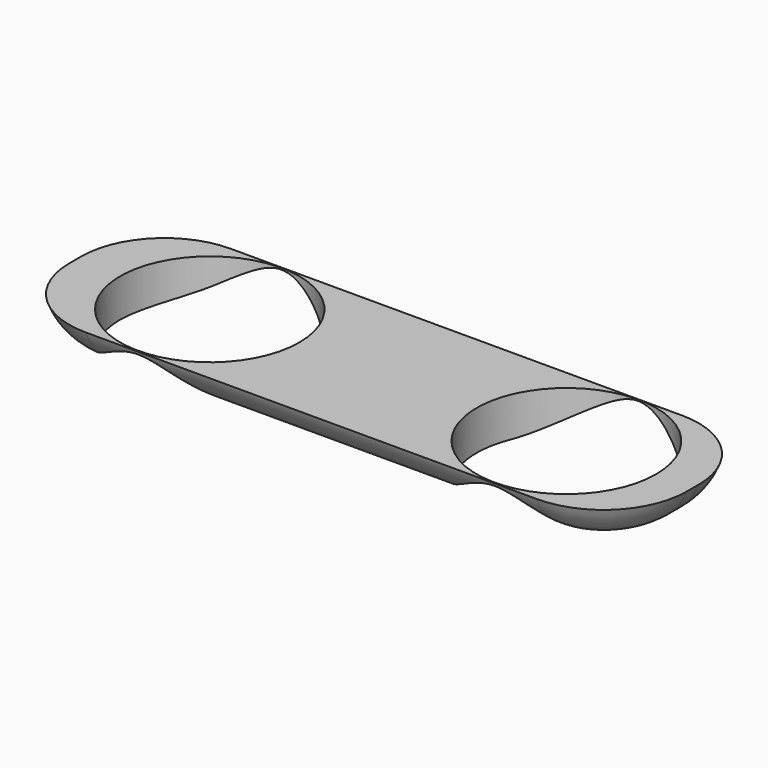
from build123d import *

# Parameters (mm, degrees)
F0_R         = 25.3224131448
F0_R_2       = 25.3609127301
F1_DEPTH     = 11.176
F2_T1_DEPTH  = 4.1998379789
F2_T3_DEPTH  = 127.4783204379
F2_T5_DEPTH  = 4.1998416744
F2_T7_DEPTH  = 127.4783167424
F2_T10_ANGLE = 90
F2_T12_ANGLE = 90
F2_T14_ANGLE = 90
F2_T16_ANGLE = 90


# Not quite as in the source:
# - a fillet or chamfer that OpenCascade refuses, or shapes differently, is made with other operations: its cross-section is extruded or revolved along the edge and cut away or added


with BuildPart() as f1:
    # F0 (on Top) → F1 (new body)
    with BuildSketch(Plane.XY):
        with BuildLine():
            Line((70.0572131213, 37.4184697866), (-57.4211036211, 37.4184697866))
            ThreePointArc((-57.4211036211, 37.4184697866), (-74.0383517658, 30.5353802358), (-80.9214413166, 13.9181320912))
            Line((-80.9214413166, 13.9181320912), (-80.9214413166, 9.7182941123))
            ThreePointArc((-80.9214413166, 9.7182941123), (-74.0383528482, -6.8989514193), (-57.4211073166, -13.7820398877))
            Line((-57.4211073166, -13.7820398877), (70.0572131213, -13.7820398877))
            ThreePointArc((70.0572131213, -13.7820398877), (86.6744586529, -6.8989514193), (93.5575471213, 9.7182941123))
            Line((93.5575471213, 9.7182941123), (93.5575471213, 13.9181357866))
            ThreePointArc((93.5575471213, 13.9181357866), (86.6744586529, 30.5353813182), (70.0572131213, 37.4184697866))
        make_face()
        with Locations((-42.9976209998, 11.9247278199)):
            Circle(F0_R, mode=Mode.SUBTRACT)
        with Locations((57.7639937401, 11.9247278199)):
            Circle(F0_R_2, mode=Mode.SUBTRACT)
    extrude(amount=F1_DEPTH)

    # F2: fillet of radius 17.1698868556 on 1 edges, made by hand

    # F2_s2 → F2_t1 (cut)
    with BuildSketch(Plane.XZ.offset(-13.9181320912)):
        with BuildLine():
            ThreePointArc((-80.9214413166, 11.176), (-74.6269133611, 3.0681250194), (-64.8317447689, 0))
            Line((-64.8317447689, 0), (-64.8317447689, -0.3433977371))
            Line((-64.8317447689, -0.3433977371), (-80.9214413166, -0.3433977371))
            Line((-80.9214413166, -0.3433977371), (-81.2648390537, 0))
            ThreePointArc((-81.2648390537, 0), (-81.2648390537, 5.588), (-81.2432352476, 11.0561222629))
            Line((-81.2432352476, 11.0561222629), (-80.9214413166, 11.176))
        make_face()
    extrude(amount=F2_T1_DEPTH, mode=Mode.SUBTRACT)

    # F2_s4 → F2_t3 (cut)
    with BuildSketch(Plane.YZ.offset(-57.4211073166)):
        with BuildLine():
            ThreePointArc((-13.7820398877, 11.176), (-7.4875119322, 3.0681250194), (2.3076566599, 0))
            Line((2.3076566599, 0), (2.3076566599, -0.3433977371))
            Line((2.3076566599, -0.3433977371), (-13.7820398877, -0.3433977371))
            Line((-13.7820398877, -0.3433977371), (-14.1254376248, 0))
            ThreePointArc((-14.1254376248, 0), (-14.1254376248, 5.588), (-14.1038338187, 11.0561222629))
            Line((-14.1038338187, 11.0561222629), (-13.7820398877, 11.176))
        make_face()
    extrude(amount=F2_T3_DEPTH, mode=Mode.SUBTRACT)

    # F2_s6 → F2_t5 (cut)
    with BuildSketch(Plane.XZ.offset(-13.9181357866)):
        with BuildLine():
            ThreePointArc((93.5575471213, 11.176), (87.2630191658, 3.0681250194), (77.4678505736, 0))
            Line((77.4678505736, 0), (77.4678505736, -0.3433977371))
            Line((77.4678505736, -0.3433977371), (93.5575471213, -0.3433977371))
            Line((93.5575471213, -0.3433977371), (93.9009448584, 0))
            ThreePointArc((93.9009448584, 0), (93.9009448584, 5.588), (93.8793410523, 11.0561222629))
            Line((93.8793410523, 11.0561222629), (93.5575471213, 11.176))
        make_face()
    extrude(amount=F2_T5_DEPTH, mode=Mode.SUBTRACT)

    # F2_s8 → F2_t7 (cut)
    with BuildSketch(Plane.YZ.offset(-57.4211036211)):
        with BuildLine():
            ThreePointArc((37.4184697866, 11.176), (31.1239418311, 3.0681250194), (21.328773239, 0))
            Line((21.328773239, 0), (21.328773239, -0.3433977371))
            Line((21.328773239, -0.3433977371), (37.4184697866, -0.3433977371))
            Line((37.4184697866, -0.3433977371), (37.7618675238, 0))
            ThreePointArc((37.7618675238, 0), (37.7618675238, 5.588), (37.7402637176, 11.0561222629))
            Line((37.7402637176, 11.0561222629), (37.4184697866, 11.176))
        make_face()
    extrude(amount=F2_T7_DEPTH, mode=Mode.SUBTRACT)

    # F2_s9 → F2_t10 (revolve, cut)
    with BuildSketch(Plane.XZ.offset(-9.7182941123)):
        with BuildLine():
            ThreePointArc((-80.9214413166, 11.176), (-74.6269133611, 3.0681250194), (-64.8317447689, 0))
            Line((-64.8317447689, 0), (-64.8317447689, -0.3433977371))
            Line((-64.8317447689, -0.3433977371), (-80.9214413166, -0.3433977371))
            Line((-80.9214413166, -0.3433977371), (-81.2648390537, 0))
            ThreePointArc((-81.2648390537, 0), (-81.2648390537, 5.588), (-81.2432352476, 11.0561222629))
            Line((-81.2432352476, 11.0561222629), (-80.9214413166, 11.176))
        make_face()
    revolve(axis=Axis((-57.4211073166, 9.7182941123, 0), (0, 0, 1)), revolution_arc=F2_T10_ANGLE, mode=Mode.SUBTRACT)

    # F2_s11 → F2_t12 (revolve, cut)
    with BuildSketch(Plane.YZ.offset(70.0572131213)):
        with BuildLine():
            ThreePointArc((-13.7820398877, 11.176), (-7.4875119322, 3.0681250194), (2.3076566599, 0))
            Line((2.3076566599, 0), (2.3076566599, -0.3433977371))
            Line((2.3076566599, -0.3433977371), (-13.7820398877, -0.3433977371))
            Line((-13.7820398877, -0.3433977371), (-14.1254376248, 0))
            ThreePointArc((-14.1254376248, 0), (-14.1254376248, 5.588), (-14.1038338187, 11.0561222629))
            Line((-14.1038338187, 11.0561222629), (-13.7820398877, 11.176))
        make_face()
    revolve(axis=Axis((70.0572131213, 9.7182941123, 0), (0, 0, 1)), revolution_arc=F2_T12_ANGLE, mode=Mode.SUBTRACT)

    # F2_s13 → F2_t14 (revolve, cut)
    with BuildSketch(Plane.XZ.offset(-13.9181357866)):
        with BuildLine():
            ThreePointArc((93.5575471213, 11.176), (87.2630191658, 3.0681250194), (77.4678505736, 0))
            Line((77.4678505736, 0), (77.4678505736, -0.3433977371))
            Line((77.4678505736, -0.3433977371), (93.5575471213, -0.3433977371))
            Line((93.5575471213, -0.3433977371), (93.9009448584, 0))
            ThreePointArc((93.9009448584, 0), (93.9009448584, 5.588), (93.8793410523, 11.0561222629))
            Line((93.8793410523, 11.0561222629), (93.5575471213, 11.176))
        make_face()
    revolve(axis=Axis((70.0572131213, 13.9181357866, 0), (0, 0, 1)), revolution_arc=F2_T14_ANGLE, mode=Mode.SUBTRACT)

    # F2_s15 → F2_t16 (revolve, cut)
    with BuildSketch(Plane.YZ.offset(-57.4211036211)):
        with BuildLine():
            ThreePointArc((37.4184697866, 11.176), (31.1239418311, 3.0681250194), (21.328773239, 0))
            Line((21.328773239, 0), (21.328773239, -0.3433977371))
            Line((21.328773239, -0.3433977371), (37.4184697866, -0.3433977371))
            Line((37.4184697866, -0.3433977371), (37.7618675238, 0))
            ThreePointArc((37.7618675238, 0), (37.7618675238, 5.588), (37.7402637176, 11.0561222629))
            Line((37.7402637176, 11.0561222629), (37.4184697866, 11.176))
        make_face()
    revolve(axis=Axis((-57.4211036211, 13.9181320912, 0), (0, 0, 1)), revolution_arc=F2_T16_ANGLE, mode=Mode.SUBTRACT)


solid = f1.part
